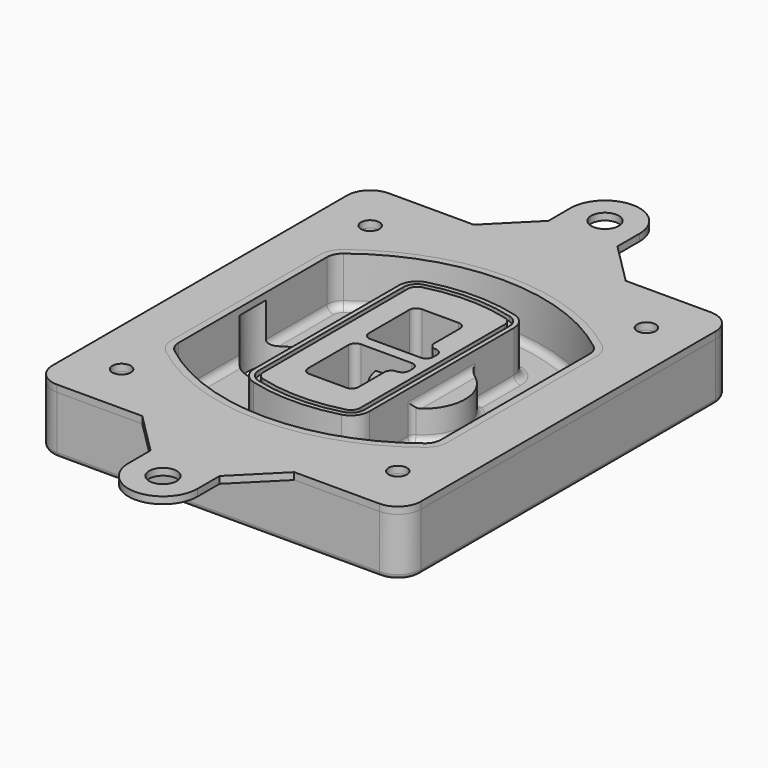
from build123d import *

# Parameters (mm, degrees)
F0_R      = 4
F1_DEPTH  = 25
F2_DEPTH  = 3
F3_DEPTH  = 18
F5_DEPTH  = 21
F6_DEPTH  = 2
F8_DEPTH  = 20
F9_DEPTH  = 16
F10_DEPTH = 25
F7_R      = 6
F7_R_2    = 4
F11_DEPTH = 6
F13_DEPTH = 9
F14_R     = 3
F15_R     = 2
F16_R     = 6
F16_R_2   = 4
F17_DEPTH = 3


with BuildPart() as f1:
    # F0 (on Top) → F1 (new body)
    with BuildSketch(Plane.XY):
        with BuildLine():
            ThreePointArc((-80, -80), (-77.0710678119, -87.0710678119), (-70, -90))
            Line((-70, -90), (70, -90))
            ThreePointArc((70, -90), (77.0710678119, -87.0710678119), (80, -80))
            Line((80, -80), (80, 80))
            ThreePointArc((80, 80), (77.0710678119, 87.0710678119), (70, 90))
            Line((70, 90), (-70, 90))
            ThreePointArc((-70, 90), (-77.0710678119, 87.0710678119), (-80, 80))
            Line((-80, 80), (-80, -80))
        make_face()
        with Locations((-60, -67.5)):
            Circle(F0_R, mode=Mode.SUBTRACT)
        with Locations((60, -67.5)):
            Circle(F0_R, mode=Mode.SUBTRACT)
        with Locations((-60, 67.5)):
            Circle(F0_R, mode=Mode.SUBTRACT)
        with BuildLine():
            ThreePointArc((-64, 40.2934422872), (-62.5820384798, 46.4328484224), (-58.6153846154, 51.3286200352))
            ThreePointArc((-58.6153846154, 51.3286200352), (0, 71.5), (58.6153846154, 51.3286200352))
            ThreePointArc((58.6153846154, 51.3286200352), (62.5820384798, 46.4328484224), (64, 40.2934422872))
            Line((64, 40.2934422872), (64, -40.2934422872))
            ThreePointArc((64, -40.2934422872), (62.5820384798, -46.4328484224), (58.6153846154, -51.3286200352))
            ThreePointArc((58.6153846154, -51.3286200352), (0, -71.5), (-58.6153846154, -51.3286200352))
            ThreePointArc((-58.6153846154, -51.3286200352), (-62.5820384798, -46.4328484224), (-64, -40.2934422872))
            Line((-64, -40.2934422872), (-64, 40.2934422872))
        make_face(mode=Mode.SUBTRACT)
        with Locations((60, 67.5)):
            Circle(F0_R, mode=Mode.SUBTRACT)
        with BuildLine():
            ThreePointArc((58.6153846154, 51.3286200352), (0, 71.5), (-58.6153846154, 51.3286200352))
            ThreePointArc((-58.6153846154, 51.3286200352), (-62.5820384798, 46.4328484224), (-64, 40.2934422872))
            Line((-64, 40.2934422872), (-64, -40.2934422872))
            ThreePointArc((-64, -40.2934422872), (-62.5820384798, -46.4328484224), (-58.6153846154, -51.3286200352))
            ThreePointArc((-58.6153846154, -51.3286200352), (0, -71.5), (58.6153846154, -51.3286200352))
            ThreePointArc((58.6153846154, -51.3286200352), (62.5820384798, -46.4328484224), (64, -40.2934422872))
            Line((64, -40.2934422872), (64, 40.2934422872))
            ThreePointArc((64, 40.2934422872), (62.5820384798, 46.4328484224), (58.6153846154, 51.3286200352))
        make_face()
        with BuildLine():
            Line((-60, -40.2934422872), (-60, 40.2934422872))
            ThreePointArc((-60, 40.2934422872), (-58.9871703427, 44.6787323838), (-56.1538461538, 48.1757121072))
            ThreePointArc((-56.1538461538, 48.1757121072), (0, 67.5), (56.1538461538, 48.1757121072))
            ThreePointArc((56.1538461538, 48.1757121072), (58.9871703427, 44.6787323838), (60, 40.2934422872))
            Line((60, 40.2934422872), (60, -40.2934422872))
            ThreePointArc((60, -40.2934422872), (58.9871703427, -44.6787323838), (56.1538461538, -48.1757121072))
            ThreePointArc((56.1538461538, -48.1757121072), (0, -67.5), (-56.1538461538, -48.1757121072))
            ThreePointArc((-56.1538461538, -48.1757121072), (-58.9871703427, -44.6787323838), (-60, -40.2934422872))
        make_face(mode=Mode.SUBTRACT)
        with BuildLine():
            ThreePointArc((-56.1538461538, 48.1757121072), (-58.9871703427, 44.6787323838), (-60, 40.2934422872))
            Line((-60, 40.2934422872), (-60, -40.2934422872))
            ThreePointArc((-60, -40.2934422872), (-58.9871703427, -44.6787323838), (-56.1538461538, -48.1757121072))
            ThreePointArc((-56.1538461538, -48.1757121072), (0, -67.5), (56.1538461538, -48.1757121072))
            ThreePointArc((56.1538461538, -48.1757121072), (58.9871703427, -44.6787323838), (60, -40.2934422872))
            Line((60, -40.2934422872), (60, 40.2934422872))
            ThreePointArc((60, 40.2934422872), (58.9871703427, 44.6787323838), (56.1538461538, 48.1757121072))
            ThreePointArc((56.1538461538, 48.1757121072), (0, 67.5), (-56.1538461538, 48.1757121072))
        make_face()
        with BuildLine():
            ThreePointArc((54.3076923077, 45.8110311612), (56.2910192399, 43.3631453548), (57, 40.2934422872))
            Line((57, 40.2934422872), (57, -40.2934422872))
            ThreePointArc((57, -40.2934422872), (56.2910192399, -43.3631453548), (54.3076923077, -45.8110311612))
            ThreePointArc((54.3076923077, -45.8110311612), (0, -64.5), (-54.3076923077, -45.8110311612))
            ThreePointArc((-54.3076923077, -45.8110311612), (-56.2910192399, -43.3631453548), (-57, -40.2934422872))
            Line((-57, -40.2934422872), (-57, 40.2934422872))
            ThreePointArc((-57, 40.2934422872), (-56.2910192399, 43.3631453548), (-54.3076923077, 45.8110311612))
            ThreePointArc((-54.3076923077, 45.8110311612), (0, 64.5), (54.3076923077, 45.8110311612))
        make_face(mode=Mode.SUBTRACT)
        with BuildLine():
            Line((57, -40.2934422872), (57, 40.2934422872))
            ThreePointArc((57, 40.2934422872), (56.2910192399, 43.3631453548), (54.3076923077, 45.8110311612))
            ThreePointArc((54.3076923077, 45.8110311612), (0, 64.5), (-54.3076923077, 45.8110311612))
            ThreePointArc((-54.3076923077, 45.8110311612), (-56.2910192399, 43.3631453548), (-57, 40.2934422872))
            Line((-57, 40.2934422872), (-57, -40.2934422872))
            ThreePointArc((-57, -40.2934422872), (-56.2910192399, -43.3631453548), (-54.3076923077, -45.8110311612))
            ThreePointArc((-54.3076923077, -45.8110311612), (0, -64.5), (54.3076923077, -45.8110311612))
            ThreePointArc((54.3076923077, -45.8110311612), (56.2910192399, -43.3631453548), (57, -40.2934422872))
        make_face()
    extrude(amount=-F1_DEPTH)

    # F0 (on Top) → F2 (join)
    with BuildSketch(Plane.XY):
        with BuildLine():
            ThreePointArc((-56.1538461538, 48.1757121072), (-58.9871703427, 44.6787323838), (-60, 40.2934422872))
            Line((-60, 40.2934422872), (-60, -40.2934422872))
            ThreePointArc((-60, -40.2934422872), (-58.9871703427, -44.6787323838), (-56.1538461538, -48.1757121072))
            ThreePointArc((-56.1538461538, -48.1757121072), (0, -67.5), (56.1538461538, -48.1757121072))
            ThreePointArc((56.1538461538, -48.1757121072), (58.9871703427, -44.6787323838), (60, -40.2934422872))
            Line((60, -40.2934422872), (60, 40.2934422872))
            ThreePointArc((60, 40.2934422872), (58.9871703427, 44.6787323838), (56.1538461538, 48.1757121072))
            ThreePointArc((56.1538461538, 48.1757121072), (0, 67.5), (-56.1538461538, 48.1757121072))
        make_face()
        with BuildLine():
            ThreePointArc((54.3076923077, 45.8110311612), (56.2910192399, 43.3631453548), (57, 40.2934422872))
            Line((57, 40.2934422872), (57, -40.2934422872))
            ThreePointArc((57, -40.2934422872), (56.2910192399, -43.3631453548), (54.3076923077, -45.8110311612))
            ThreePointArc((54.3076923077, -45.8110311612), (0, -64.5), (-54.3076923077, -45.8110311612))
            ThreePointArc((-54.3076923077, -45.8110311612), (-56.2910192399, -43.3631453548), (-57, -40.2934422872))
            Line((-57, -40.2934422872), (-57, 40.2934422872))
            ThreePointArc((-57, 40.2934422872), (-56.2910192399, 43.3631453548), (-54.3076923077, 45.8110311612))
            ThreePointArc((-54.3076923077, 45.8110311612), (0, 64.5), (54.3076923077, 45.8110311612))
        make_face(mode=Mode.SUBTRACT)
    extrude(amount=F2_DEPTH)

    # F0 (on Top) → F3 (cut)
    with BuildSketch(Plane.XY):
        with BuildLine():
            Line((57, -40.2934422872), (57, 40.2934422872))
            ThreePointArc((57, 40.2934422872), (56.2910192399, 43.3631453548), (54.3076923077, 45.8110311612))
            ThreePointArc((54.3076923077, 45.8110311612), (0, 64.5), (-54.3076923077, 45.8110311612))
            ThreePointArc((-54.3076923077, 45.8110311612), (-56.2910192399, 43.3631453548), (-57, 40.2934422872))
            Line((-57, 40.2934422872), (-57, -40.2934422872))
            ThreePointArc((-57, -40.2934422872), (-56.2910192399, -43.3631453548), (-54.3076923077, -45.8110311612))
            ThreePointArc((-54.3076923077, -45.8110311612), (0, -64.5), (54.3076923077, -45.8110311612))
            ThreePointArc((54.3076923077, -45.8110311612), (56.2910192399, -43.3631453548), (57, -40.2934422872))
        make_face()
    extrude(amount=-F3_DEPTH, mode=Mode.SUBTRACT)

    # F4 (on face) → F5 (join, through all)
    with BuildSketch(Plane.XY.offset(3)):
        with BuildLine():
            ThreePointArc((-25, -39.2465276821), (-23.3511545998, -44.1109737193), (-19.0842911877, -46.9702398883))
            ThreePointArc((-19.0842911877, -46.9702398883), (0, -49.5), (19.0842911877, -46.9702398883))
            ThreePointArc((19.0842911877, -46.9702398883), (23.3511545998, -44.1109737193), (25, -39.2465276821))
            Line((25, -39.2465276821), (25, 39.2465276821))
            ThreePointArc((25, 39.2465276821), (23.3511545998, 44.1109737193), (19.0842911877, 46.9702398883))
            ThreePointArc((19.0842911877, 46.9702398883), (0, 49.5), (-19.0842911877, 46.9702398883))
            ThreePointArc((-19.0842911877, 46.9702398883), (-23.3511545998, 44.1109737193), (-25, 39.2465276821))
            Line((-25, 39.2465276821), (-25, -39.2465276821))
        make_face()
        with BuildLine():
            ThreePointArc((18.5632183908, 45.0393118368), (21.7633659499, 42.89486221), (23, 39.2465276821))
            Line((23, 39.2465276821), (23, -39.2465276821))
            ThreePointArc((23, -39.2465276821), (21.7633659499, -42.89486221), (18.5632183908, -45.0393118368))
            ThreePointArc((18.5632183908, -45.0393118368), (0, -47.5), (-18.5632183908, -45.0393118368))
            ThreePointArc((-18.5632183908, -45.0393118368), (-21.7633659499, -42.89486221), (-23, -39.2465276821))
            Line((-23, -39.2465276821), (-23, 39.2465276821))
            ThreePointArc((-23, 39.2465276821), (-21.7633659499, 42.89486221), (-18.5632183908, 45.0393118368))
            ThreePointArc((-18.5632183908, 45.0393118368), (0, 47.5), (18.5632183908, 45.0393118368))
        make_face(mode=Mode.SUBTRACT)
        with BuildLine():
            Line((23, -39.2465276821), (23, 39.2465276821))
            ThreePointArc((23, 39.2465276821), (21.7633659499, 42.89486221), (18.5632183908, 45.0393118368))
            ThreePointArc((18.5632183908, 45.0393118368), (0, 47.5), (-18.5632183908, 45.0393118368))
            ThreePointArc((-18.5632183908, 45.0393118368), (-21.7633659499, 42.89486221), (-23, 39.2465276821))
            Line((-23, 39.2465276821), (-23, -39.2465276821))
            ThreePointArc((-23, -39.2465276821), (-21.7633659499, -42.89486221), (-18.5632183908, -45.0393118368))
            ThreePointArc((-18.5632183908, -45.0393118368), (0, -47.5), (18.5632183908, -45.0393118368))
            ThreePointArc((18.5632183908, -45.0393118368), (21.7633659499, -42.89486221), (23, -39.2465276821))
        make_face()
        with BuildLine():
            ThreePointArc((18.0421455939, 43.1083837852), (20.1755772999, 41.6787507007), (21, 39.2465276821))
            Line((21, 39.2465276821), (21, -39.2465276821))
            ThreePointArc((21, -39.2465276821), (20.1755772999, -41.6787507007), (18.0421455939, -43.1083837852))
            ThreePointArc((18.0421455939, -43.1083837852), (0, -45.5), (-18.0421455939, -43.1083837852))
            ThreePointArc((-18.0421455939, -43.1083837852), (-20.1755772999, -41.6787507007), (-21, -39.2465276821))
            Line((-21, -39.2465276821), (-21, 39.2465276821))
            ThreePointArc((-21, 39.2465276821), (-20.1755772999, 41.6787507007), (-18.0421455939, 43.1083837852))
            ThreePointArc((-18.0421455939, 43.1083837852), (0, 45.5), (18.0421455939, 43.1083837852))
        make_face(mode=Mode.SUBTRACT)
        with BuildLine():
            Line((21, -39.2465276821), (21, 39.2465276821))
            ThreePointArc((21, 39.2465276821), (20.1755772999, 41.6787507007), (18.0421455939, 43.1083837852))
            ThreePointArc((18.0421455939, 43.1083837852), (0, 45.5), (-18.0421455939, 43.1083837852))
            ThreePointArc((-18.0421455939, 43.1083837852), (-20.1755772999, 41.6787507007), (-21, 39.2465276821))
            Line((-21, 39.2465276821), (-21, -39.2465276821))
            ThreePointArc((-21, -39.2465276821), (-20.1755772999, -41.6787507007), (-18.0421455939, -43.1083837852))
            ThreePointArc((-18.0421455939, -43.1083837852), (0, -45.5), (18.0421455939, -43.1083837852))
            ThreePointArc((18.0421455939, -43.1083837852), (20.1755772999, -41.6787507007), (21, -39.2465276821))
        make_face()
        with BuildLine():
            Line((-8, -2.5), (14, -2.5))
            ThreePointArc((14, -2.5), (16.1213203436, -3.3786796564), (17, -5.5))
            Line((17, -5.5), (17, -7.5))
            ThreePointArc((17, -7.5), (16.1213203436, -9.6213203436), (14, -10.5))
            ThreePointArc((14, -10.5), (11.8786796564, -11.3786796564), (11, -13.5))
            Line((11, -13.5), (11, -27.5))
            ThreePointArc((11, -27.5), (10.1213203436, -29.6213203436), (8, -30.5))
            Line((8, -30.5), (-8, -30.5))
            ThreePointArc((-8, -30.5), (-10.1213203436, -29.6213203436), (-11, -27.5))
            Line((-11, -27.5), (-11, -5.5))
            ThreePointArc((-11, -5.5), (-10.1213203436, -3.3786796564), (-8, -2.5))
        make_face(mode=Mode.SUBTRACT)
        with BuildLine():
            ThreePointArc((-8, 2.5), (-10.1213203436, 3.3786796564), (-11, 5.5))
            Line((-11, 5.5), (-11, 27.5))
            ThreePointArc((-11, 27.5), (-10.1213203436, 29.6213203436), (-8, 30.5))
            Line((-8, 30.5), (8, 30.5))
            ThreePointArc((8, 30.5), (10.1213203436, 29.6213203436), (11, 27.5))
            Line((11, 27.5), (11, 13.5))
            ThreePointArc((11, 13.5), (11.8786796564, 11.3786796564), (14, 10.5))
            ThreePointArc((14, 10.5), (16.1213203436, 9.6213203436), (17, 7.5))
            Line((17, 7.5), (17, 5.5))
            ThreePointArc((17, 5.5), (16.1213203436, 3.3786796564), (14, 2.5))
            Line((14, 2.5), (-8, 2.5))
        make_face(mode=Mode.SUBTRACT)
    extrude(amount=-F5_DEPTH)

    # F4 (on face) → F6 (cut)
    with BuildSketch(Plane.XY.offset(3)):
        with BuildLine():
            Line((23, -39.2465276821), (23, 39.2465276821))
            ThreePointArc((23, 39.2465276821), (21.7633659499, 42.89486221), (18.5632183908, 45.0393118368))
            ThreePointArc((18.5632183908, 45.0393118368), (0, 47.5), (-18.5632183908, 45.0393118368))
            ThreePointArc((-18.5632183908, 45.0393118368), (-21.7633659499, 42.89486221), (-23, 39.2465276821))
            Line((-23, 39.2465276821), (-23, -39.2465276821))
            ThreePointArc((-23, -39.2465276821), (-21.7633659499, -42.89486221), (-18.5632183908, -45.0393118368))
            ThreePointArc((-18.5632183908, -45.0393118368), (0, -47.5), (18.5632183908, -45.0393118368))
            ThreePointArc((18.5632183908, -45.0393118368), (21.7633659499, -42.89486221), (23, -39.2465276821))
        make_face()
        with BuildLine():
            ThreePointArc((18.0421455939, 43.1083837852), (20.1755772999, 41.6787507007), (21, 39.2465276821))
            Line((21, 39.2465276821), (21, -39.2465276821))
            ThreePointArc((21, -39.2465276821), (20.1755772999, -41.6787507007), (18.0421455939, -43.1083837852))
            ThreePointArc((18.0421455939, -43.1083837852), (0, -45.5), (-18.0421455939, -43.1083837852))
            ThreePointArc((-18.0421455939, -43.1083837852), (-20.1755772999, -41.6787507007), (-21, -39.2465276821))
            Line((-21, -39.2465276821), (-21, 39.2465276821))
            ThreePointArc((-21, 39.2465276821), (-20.1755772999, 41.6787507007), (-18.0421455939, 43.1083837852))
            ThreePointArc((-18.0421455939, 43.1083837852), (0, 45.5), (18.0421455939, 43.1083837852))
        make_face(mode=Mode.SUBTRACT)
    extrude(amount=-F6_DEPTH, mode=Mode.SUBTRACT)

    # F7 (on face) → F8 (join)
    with BuildSketch(Plane(origin=(0, 0, -25), x_dir=(1, 0, 0), z_dir=(0, 0, -1))):
        with BuildLine():
            ThreePointArc((3.28842436, 0), (16.7567035675, 13.4682792075), (30.224982775, 0))
            Line((30.224982775, 0), (35.224982775, 0))
            ThreePointArc((35.224982775, 0), (16.7567035675, 18.4682792075), (-1.71157564, 0))
            Line((-1.71157564, 0), (3.28842436, 0))
        make_face()
        with BuildLine():
            Line((3.28842436, 0), (30.224982775, 0))
            ThreePointArc((30.224982775, 0), (16.7567035675, 13.4682792075), (3.28842436, 0))
        make_face()
        with BuildLine():
            ThreePointArc((3.28842436, 0), (16.7567035675, -13.4682792075), (30.224982775, 0))
            Line((30.224982775, 0), (3.28842436, 0))
        make_face()
        with BuildLine():
            Line((35.224982775, 0), (30.224982775, 0))
            ThreePointArc((30.224982775, 0), (16.7567035675, -13.4682792075), (3.28842436, 0))
            Line((3.28842436, 0), (-1.71157564, 0))
            ThreePointArc((-1.71157564, 0), (16.7567035675, -18.4682792075), (35.224982775, 0))
        make_face()
    extrude(amount=-F8_DEPTH)

    # F7 (on face) → F9 (cut)
    with BuildSketch(Plane(origin=(0, 0, -25), x_dir=(1, 0, 0), z_dir=(0, 0, -1))):
        with BuildLine():
            Line((3.28842436, 0), (30.224982775, 0))
            ThreePointArc((30.224982775, 0), (16.7567035675, 13.4682792075), (3.28842436, 0))
        make_face()
        with BuildLine():
            ThreePointArc((3.28842436, 0), (16.7567035675, -13.4682792075), (30.224982775, 0))
            Line((30.224982775, 0), (3.28842436, 0))
        make_face()
    extrude(amount=-F9_DEPTH, mode=Mode.SUBTRACT)

    # F7 (on face) → F10 (cut)
    with BuildSketch(Plane(origin=(0, 0, -25), x_dir=(1, 0, 0), z_dir=(0, 0, -1))):
        with BuildLine():
            Line((-59.0318229325, 0), (-32.0952645175, 0))
            ThreePointArc((-32.0952645175, 0), (-45.563543725, 13.4682792075), (-59.0318229325, 0))
        make_face()
        with BuildLine():
            ThreePointArc((-59.0318229325, 0), (-45.563543725, -13.4682792075), (-32.0952645175, 0))
            Line((-32.0952645175, 0), (-59.0318229325, 0))
        make_face()
    extrude(amount=-F10_DEPTH, mode=Mode.SUBTRACT)

    # F7 (on face) → F11 (cut)
    with BuildSketch(Plane(origin=(0, 0, -25), x_dir=(1, 0, 0), z_dir=(0, 0, -1))):
        with Locations((60, -67.5)):
            Circle(F7_R)
        with Locations((60, -67.5)):
            Circle(F7_R_2, mode=Mode.SUBTRACT)
        with Locations((-60, -67.5)):
            Circle(F7_R)
        with Locations((-60, -67.5)):
            Circle(F7_R_2, mode=Mode.SUBTRACT)
        with Locations((-60, 67.5)):
            Circle(F7_R)
        with Locations((-60, 67.5)):
            Circle(F7_R_2, mode=Mode.SUBTRACT)
        with Locations((60, 67.5)):
            Circle(F7_R)
        with Locations((60, 67.5)):
            Circle(F7_R_2, mode=Mode.SUBTRACT)
    extrude(amount=-F11_DEPTH, mode=Mode.SUBTRACT)

    # F12 (on face) → F13 (cut, through all)
    with BuildSketch(Plane(origin=(0, 0, -9), x_dir=(1, 0, 0), z_dir=(0, 0, -1))):
        with BuildLine():
            Line((11, 13.5), (11, 17.5481537753))
            ThreePointArc((11, 17.5481537753), (2.5696536419, 11.8239143813), (-1.5415842455, 2.5))
            Line((-1.5415842455, 2.5), (3.5224848595, 2.5))
            ThreePointArc((3.5224848595, 2.5), (6.1857188154, 8.3455872281), (11.2536447004, 12.2927168648))
            ThreePointArc((11.2536447004, 12.2927168648), (11.0640958889, 12.8831798879), (11, 13.5))
        make_face()
        with BuildLine():
            ThreePointArc((11.2536447004, -12.2927168648), (6.1857188154, -8.3455872281), (3.5224848595, -2.5))
            Line((3.5224848595, -2.5), (-1.5415842455, -2.5))
            ThreePointArc((-1.5415842455, -2.5), (2.5696536419, -11.8239143813), (11, -17.5481537753))
            Line((11, -17.5481537753), (11, -13.5))
            ThreePointArc((11, -13.5), (11.0640958889, -12.8831798879), (11.2536447004, -12.2927168648))
        make_face()
        with BuildLine():
            ThreePointArc((11.2536447004, 12.2927168648), (6.1857188154, 8.3455872281), (3.5224848595, 2.5))
            Line((3.5224848595, 2.5), (14, 2.5))
            ThreePointArc((14, 2.5), (16.1213203436, 3.3786796564), (17, 5.5))
            Line((17, 5.5), (17, 7.5))
            ThreePointArc((17, 7.5), (16.1213203436, 9.6213203436), (14, 10.5))
            ThreePointArc((14, 10.5), (12.3601599782, 10.9878446101), (11.2536447004, 12.2927168648))
        make_face()
        with BuildLine():
            Line((14, -2.5), (3.5224848595, -2.5))
            ThreePointArc((3.5224848595, -2.5), (6.1857188154, -8.3455872281), (11.2536447004, -12.2927168648))
            ThreePointArc((11.2536447004, -12.2927168648), (12.3601599782, -10.9878446101), (14, -10.5))
            ThreePointArc((14, -10.5), (16.1213203436, -9.6213203436), (17, -7.5))
            Line((17, -7.5), (17, -5.5))
            ThreePointArc((17, -5.5), (16.1213203436, -3.3786796564), (14, -2.5))
        make_face()
    extrude(amount=F13_DEPTH, mode=Mode.SUBTRACT)

    # F14
    f14_edges = [f1.edges().sort_by_distance(p)[0] for p in [
        (-57, -23.703476, -18),
        (-57, 23.703476, -18),
        (25, 0, -5),
        (25, 16.526506, -11.5),
        (25, -16.526506, -11.5),
        (25, -27.886517, -18),
        (35.224983, 0, -18),
    ]]
    fillet(f14_edges, radius=F14_R)

    # F15
    f15_edges = [f1.edges().sort_by_distance(p)[0] for p in [
        (0, -90, -25),
    ]]
    fillet(f15_edges, radius=F15_R)


with BuildPart() as f17:
    # F16 (on face) → F17 (new body, through all)
    with BuildSketch(Plane.XY):
        with BuildLine():
            Line((33, -90), (-33, -90))
            Line((-33, -90), (-15, -108))
            Line((-15, -108), (-15, -120))
            ThreePointArc((-15, -120), (0, -135), (15, -120))
            Line((15, -120), (15, -108))
            Line((15, -108), (33, -90))
        make_face()
        with Locations((0, -120)):
            Circle(F16_R, mode=Mode.SUBTRACT)
        with BuildLine():
            ThreePointArc((15, 120), (0, 135), (-15, 120))
            Line((-15, 120), (-15, 108))
            Line((-15, 108), (-33, 90))
            Line((-33, 90), (33, 90))
            Line((33, 90), (15, 108))
            Line((15, 108), (15, 120))
        make_face()
        with Locations((0, 120)):
            Circle(F16_R, mode=Mode.SUBTRACT)
        with BuildLine():
            Line((33, 90), (-33, 90))
            Line((-33, 90), (-70, 90))
            ThreePointArc((-70, 90), (-77.0710678119, 87.0710678119), (-80, 80))
            Line((-80, 80), (-80, -80))
            ThreePointArc((-80, -80), (-77.0710678119, -87.0710678119), (-70, -90))
            Line((-70, -90), (-33, -90))
            Line((-33, -90), (33, -90))
            Line((33, -90), (70, -90))
            ThreePointArc((70, -90), (77.0710678119, -87.0710678119), (80, -80))
            Line((80, -80), (80, 80))
            ThreePointArc((80, 80), (77.0710678119, 87.0710678119), (70, 90))
            Line((70, 90), (33, 90))
        make_face()
        with Locations((-60, -67.5)):
            Circle(F16_R_2, mode=Mode.SUBTRACT)
        with Locations((60, -67.5)):
            Circle(F16_R_2, mode=Mode.SUBTRACT)
        with Locations((-60, 67.5)):
            Circle(F16_R_2, mode=Mode.SUBTRACT)
        with BuildLine():
            ThreePointArc((-60, 40.2934422872), (-58.9871703427, 44.6787323838), (-56.1538461538, 48.1757121072))
            ThreePointArc((-56.1538461538, 48.1757121072), (0, 67.5), (56.1538461538, 48.1757121072))
            ThreePointArc((56.1538461538, 48.1757121072), (58.9871703427, 44.6787323838), (60, 40.2934422872))
            Line((60, 40.2934422872), (60, -40.2934422872))
            ThreePointArc((60, -40.2934422872), (58.9871703427, -44.6787323838), (56.1538461538, -48.1757121072))
            ThreePointArc((56.1538461538, -48.1757121072), (0, -67.5), (-56.1538461538, -48.1757121072))
            ThreePointArc((-56.1538461538, -48.1757121072), (-58.9871703427, -44.6787323838), (-60, -40.2934422872))
            Line((-60, -40.2934422872), (-60, 40.2934422872))
        make_face(mode=Mode.SUBTRACT)
        with Locations((60, 67.5)):
            Circle(F16_R_2, mode=Mode.SUBTRACT)
    extrude(amount=F17_DEPTH)


solid = Compound([f1.part, f17.part])
